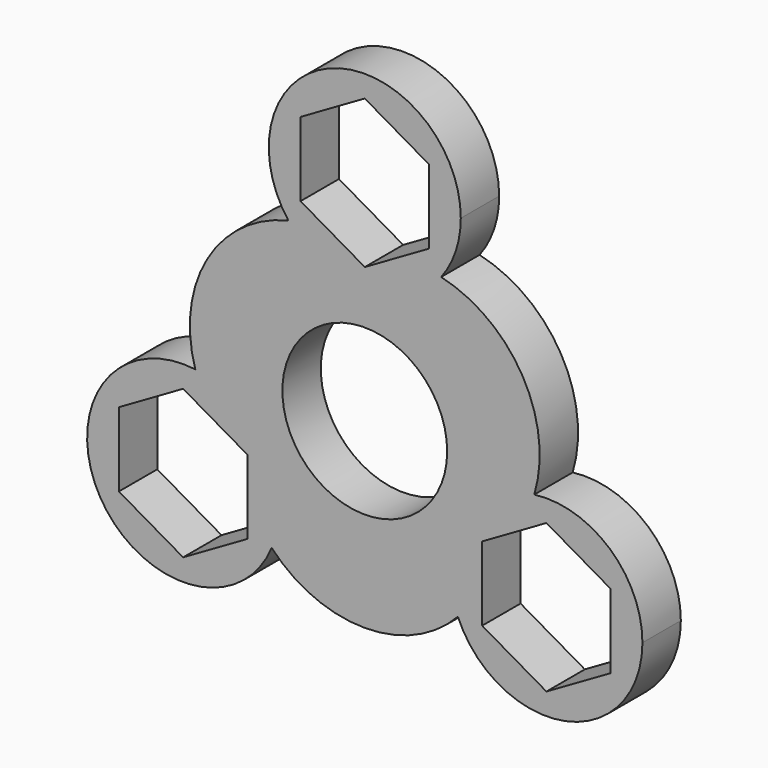
from build123d import *

# Parameters (mm, degrees)
F0_R           = 10.9
F1_DEPTH       = 6.35
F2_TEXT_SIZE   = 5.5377927816
F2_TEXT_SIZE_2 = 5.9069781047
F3_DEPTH       = 1.27


# Not quite as in the source:
# - Text() gives the source's letters only with a copy of the font that has no kerning and outlines rounded to 1/6400 em; it was checked with that copy


with BuildPart() as f1:
    # F0 (on Front) → F1 (new body)
    with BuildSketch(Plane.XZ):
        with BuildLine():
            ThreePointArc((10.1067624731, 20.0575860915), (12.0342403875, 23.6900952858), (12.7, 27.7480576187))
            ThreePointArc((12.7, 27.7480576187), (-4.0579623329, 39.7822980062), (-10.1067624731, 20.0575860915))
            ThreePointArc((-10.1067624731, 20.0575860915), (0, 15.0480576187), (10.1067624731, 20.0575860915))
        make_face()
        Polygon((0, 17.9331030425), (-8.5, 22.8405803306), (-8.5, 32.6555349068), (0, 37.563012195), (8.5, 32.6555349068), (8.5, 22.8405803306), align=None, mode=Mode.SUBTRACT)
        with BuildLine():
            ThreePointArc((10.1067624731, 20.0575860915), (0, 15.0480576187), (-10.1067624731, 20.0575860915))
            ThreePointArc((-10.1067624731, 20.0575860915), (-20.8691640461, 12.0488174798), (-22.4237603304, -1.276079994))
            ThreePointArc((-22.4237603304, -1.276079994), (-14.4991041418, -5.481052085), (-11.3305228035, -13.8740288094))
            ThreePointArc((-11.3305228035, -13.8740288094), (-11.5795837462, -16.3768505352), (-12.3169978572, -18.7815060975))
            ThreePointArc((-12.3169978572, -18.7815060975), (0, -24.0976349596), (12.3169978572, -18.7815060975))
            ThreePointArc((12.3169978572, -18.7815060975), (13.0320001754, -7.5240288094), (22.4237603304, -1.276079994))
            ThreePointArc((22.4237603304, -1.276079994), (20.8691640461, 12.0488174798), (10.1067624731, 20.0575860915))
        make_face()
        Circle(F0_R, mode=Mode.SUBTRACT)
        with BuildLine():
            ThreePointArc((-11.3305228035, -13.8740288094), (-14.4991041418, -5.481052085), (-22.4237603304, -1.276079994))
            ThreePointArc((-22.4237603304, -1.276079994), (-35.0290454316, -20.2240288094), (-12.3169978572, -18.7815060975))
            ThreePointArc((-12.3169978572, -18.7815060975), (-11.5795837462, -16.3768505352), (-11.3305228035, -13.8740288094))
        make_face()
        Polygon((-24.0305228035, -4.0590742331), (-15.5305228035, -8.9665515213), (-15.5305228035, -18.7815060975), (-24.0305228035, -23.6889833856), (-32.5305228035, -18.7815060975), (-32.5305228035, -8.9665515213), align=None, mode=Mode.SUBTRACT)
        with BuildLine():
            ThreePointArc((36.7305228035, -13.8740288094), (32.4234995279, -4.3426101477), (22.4237603304, -1.276079994))
            ThreePointArc((22.4237603304, -1.276079994), (13.0320001754, -7.5240288094), (12.3169978572, -18.7815060975))
            ThreePointArc((12.3169978572, -18.7815060975), (26.5333445293, -26.3249678667), (36.7305228035, -13.8740288094))
        make_face()
        Polygon((15.5305228035, -8.9665515213), (24.0305228035, -4.0590742331), (32.5305228035, -8.9665515213), (32.5305228035, -18.7815060975), (24.0305228035, -23.6889833856), (15.5305228035, -18.7815060975), align=None, mode=Mode.SUBTRACT)
    extrude(amount=F1_DEPTH)

    # F2 (on face) → F3 (cut)
    with BuildSketch(Plane(origin=(0, 0, 0), x_dir=(-1, 0, 0), z_dir=(0, 1, 0))):
        with Locations((-7.9956209685, -19.3126294762)):
            Text('Fidget', F2_TEXT_SIZE, font='Open Sans', text_align=(TextAlign.LEFT, TextAlign.BOTTOM))
        with Locations((-5.9143602848, 12.2938947752)):
            Text('Frog', F2_TEXT_SIZE_2, font='Open Sans', text_align=(TextAlign.LEFT, TextAlign.BOTTOM))
    extrude(amount=-F3_DEPTH, mode=Mode.SUBTRACT)


solid = f1.part
